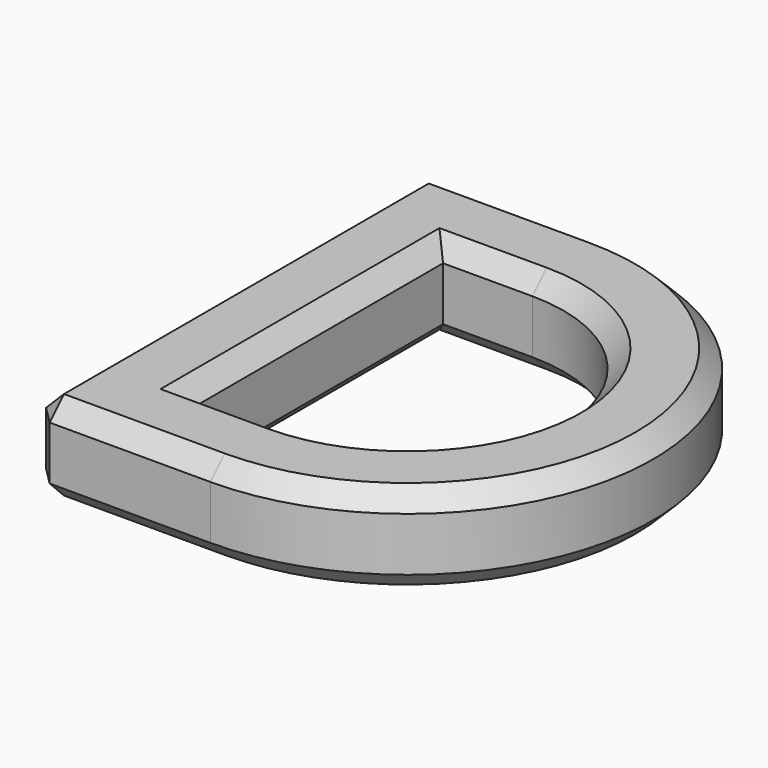
from build123d import *

# Parameters (mm, degrees)
F1_DEPTH = 2
F2_SIZE  = 0.4


# Not quite as in the source:
# - a feature names something its author has since deleted; it is built from what else it names


with BuildPart() as f1:
    # F0 (on Top) → F1 (new body)
    with BuildSketch(Plane.XY):
        with BuildLine():
            Line((-8.3299736083, -24.3851770833), (-12.3299736083, -24.3851770833))
            Line((-12.3299736083, -24.3851770833), (-12.3299736083, -35.3851770833))
            Line((-12.3299736083, -35.3851770833), (-8.3299736083, -35.3851770833))
            ThreePointArc((-8.3299736083, -35.3851770833), (-2.8299736083, -29.8851770833), (-8.3299736083, -24.3851770833))
        make_face()
        with BuildLine():
            Line((-10.3299736083, -33.3851770833), (-10.3299736083, -26.3851770833))
            Line((-10.3299736083, -26.3851770833), (-8.3299736083, -26.3851770833))
            ThreePointArc((-8.3299736083, -26.3851770833), (-4.8299736083, -29.8851770833), (-8.3299736083, -33.3851770833))
            Line((-8.3299736083, -33.3851770833), (-10.3299736083, -33.3851770833))
        make_face(mode=Mode.SUBTRACT)
    extrude(amount=F1_DEPTH)

    # F2
    f2_edges = [f1.edges().sort_by_distance(p)[0] for p in [
        (-9.329974, -33.385177, 2),
        (-10.329974, -29.885177, 2),
        (-9.329974, -26.385177, 2),
        (-10.329974, -35.385177, 2),
        (-12.329974, -29.885177, 2),
        (-12.329974, -35.385177, 1),
        (-10.329974, -24.385177, 2),
        (-12.329974, -24.385177, 1),
        (-12.329974, -29.885177, 0),
        (-10.329974, -29.885177, 0),
        (-9.329974, -26.385177, 0),
        (-10.329974, -24.385177, 0),
        (-9.329974, -33.385177, 0),
        (-10.329974, -35.385177, 0),
        (-2.829974, -29.885177, 0),
        (-2.829974, -29.885177, 2),
        (-4.829974, -29.885177, 0),
        (-4.829974, -29.885177, 2),
    ]]
    chamfer(f2_edges, length=F2_SIZE)


solid = f1.part
